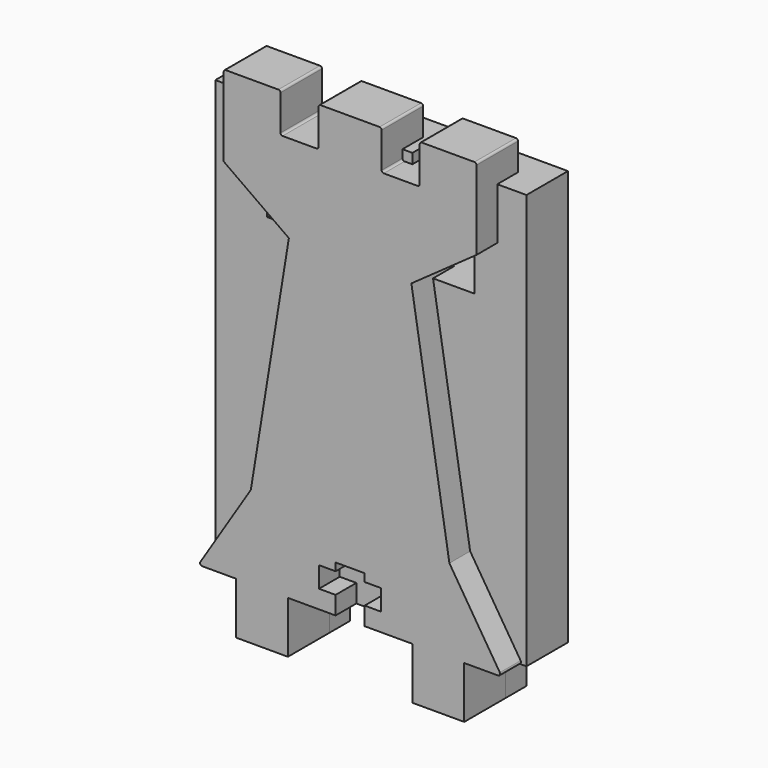
from build123d import *

# Parameters (mm, degrees)
F1_DEPTH      = 3.175
F1_DEPTH_BACK = 3.175
F2_W          = 7.62
F2_H          = 12.7
F3_DEPTH      = 25.4
F5_DEPTH      = 6.35
F7_DEPTH      = 25.4


with BuildPart() as f1:
    # F0 (on Front) → F1 (new body, two sides)
    with BuildSketch(Plane.XZ) as f1_sk:
        Polygon((-7.62, 0), (-6.35, 0), (6.35, 0), (7.62, 0), (7.62, -6.35), (13.97, -6.35), (13.97, 0), (19.05, 0), (19.05, 50.8), (-19.05, 50.8), (-19.05, 0), (-13.97, 0), (-13.97, -6.35), (-7.62, -6.35), align=None)
    extrude(amount=F1_DEPTH)
    extrude(f1_sk.sketch, amount=-F1_DEPTH_BACK)

    # F2 (on face) → F3 (cut)
    with BuildSketch(Plane.XZ.offset(3.175)):
        with Locations((-8.89, 44.45)):
            Rectangle(F2_W, F2_H)
        with Locations((8.89, 44.45)):
            Rectangle(F2_W, F2_H)
    extrude(amount=-F3_DEPTH, mode=Mode.SUBTRACT)


with BuildPart() as f5:
    # F4 (on Front) → F5 (new body)
    with BuildSketch(Plane.XZ):
        with BuildLine():
            ThreePointArc((-18.3346545666, 0.3897204487), (-18.342428457, 0.1314377586), (-18.1199548699, 0))
            Line((-18.1199548699, 0), (-13.97, 0))
            Line((-13.97, 0), (-13.97, -6.35))
            Line((-13.97, -6.35), (-7.62, -6.35))
            Line((-7.62, -6.35), (-7.62, 0))
            Line((-7.62, 0), (7.62, 0))
            Line((7.62, 0), (7.62, -6.35))
            Line((7.62, -6.35), (13.97, -6.35))
            Line((13.97, -6.35), (13.97, 0))
            Line((13.97, 0), (18.1199548699, 0))
            ThreePointArc((18.1199548699, 0), (18.342428457, 0.1314377586), (18.3346545666, 0.3897204487))
            Line((18.3346545666, 0.3897204487), (12.1539290994, 10.167170316))
            Line((12.1539290994, 10.167170316), (7.4985641986, 38.8113629378))
            Line((7.4985641986, 38.8113629378), (15.4756298289, 44.474443851))
            Line((15.4756298289, 44.474443851), (15.4756298289, 54.1500687382))
            ThreePointArc((15.4756298289, 54.1500687382), (15.4012349513, 54.3296738606), (15.2216298289, 54.4040687382))
            Line((15.2216298289, 54.4040687382), (8.7779075124, 54.4040687382))
            ThreePointArc((8.7779075124, 54.4040687382), (8.59830239, 54.3296738606), (8.5239075124, 54.1500687382))
            Line((8.5239075124, 54.1500687382), (8.5239075124, 49.8228915253))
            ThreePointArc((8.5239075124, 49.8228915253), (8.4495126348, 49.6432864028), (8.2699075124, 49.5688915253))
            Line((8.2699075124, 49.5688915253), (4.1183283769, 49.5688915253))
            ThreePointArc((4.1183283769, 49.5688915253), (3.9387232545, 49.6432864028), (3.8643283769, 49.8228915253))
            Line((3.8643283769, 49.8228915253), (3.8643283769, 54.1500687382))
            ThreePointArc((3.8643283769, 54.1500687382), (3.7899334994, 54.3296738606), (3.6103283769, 54.4040687382))
            Line((3.6103283769, 54.4040687382), (0, 54.4040687382))
            Line((0, 54.4040687382), (-3.6103283769, 54.4040687382))
            ThreePointArc((-3.6103283769, 54.4040687382), (-3.7899334994, 54.3296738606), (-3.8643283769, 54.1500687382))
            Line((-3.8643283769, 54.1500687382), (-3.8643283769, 49.8228915253))
            ThreePointArc((-3.8643283769, 49.8228915253), (-3.9387232545, 49.6432864028), (-4.1183283769, 49.5688915253))
            Line((-4.1183283769, 49.5688915253), (-8.2699075124, 49.5688915253))
            ThreePointArc((-8.2699075124, 49.5688915253), (-8.4495126348, 49.6432864028), (-8.5239075124, 49.8228915253))
            Line((-8.5239075124, 49.8228915253), (-8.5239075124, 54.1500687382))
            ThreePointArc((-8.5239075124, 54.1500687382), (-8.59830239, 54.3296738606), (-8.7779075124, 54.4040687382))
            Line((-8.7779075124, 54.4040687382), (-15.2216298289, 54.4040687382))
            ThreePointArc((-15.2216298289, 54.4040687382), (-15.4012349513, 54.3296738606), (-15.4756298289, 54.1500687382))
            Line((-15.4756298289, 54.1500687382), (-15.4756298289, 44.474443851))
            Line((-15.4756298289, 44.474443851), (-7.4985641986, 38.8113629378))
            Line((-7.4985641986, 38.8113629378), (-12.1539290994, 10.167170316))
            Line((-12.1539290994, 10.167170316), (-18.3346545666, 0.3897204487))
        make_face()
    extrude(amount=F5_DEPTH)

    # F6 (on Front) → F7 (cut)
    with BuildSketch(Plane.XZ):
        Polygon((1.778, 5.715), (-1.778, 5.715), (-1.778, 4.7625), (-3.81, 4.7625), (-3.81, 2.2225), (-1.778, 2.2225), (-1.778, 0), (1.778, 0), (1.778, 2.2225), (3.81, 2.2225), (3.81, 4.7625), (1.778, 4.7625), align=None)
    extrude(amount=F7_DEPTH, mode=Mode.SUBTRACT)


solid = Compound([f1.part, f5.part])
